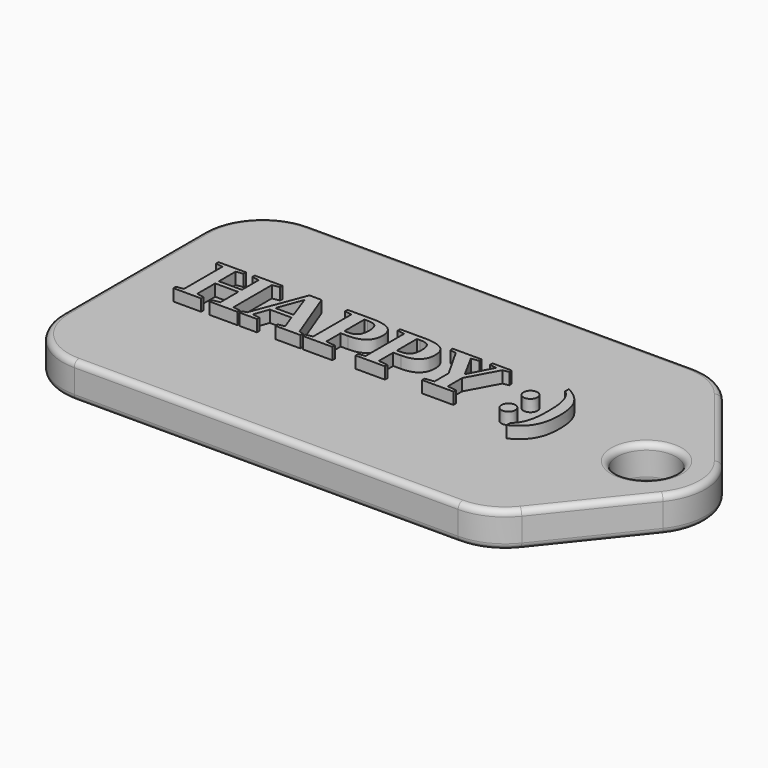
from build123d import *

# Parameters (mm, degrees)
F1_DEPTH     = 3
F2_R         = 5
F4_D         = 5
F5_R         = 5
F6_R         = 0.5
F7_TEXT_SIZE = 7.3078691558
F8_DEPTH     = 1


# Not quite as in the source:
# - Text() gives the source's letters only with a copy of the font that has no kerning and outlines rounded to 1/6400 em; it was checked with that copy


with BuildPart() as f1:
    # F0 (on Top) → F1 (new body)
    with BuildSketch(Plane.XY):
        Polygon((20, 12.5), (-20, 12.5), (-20, -12.5), (20, -12.5), (30, 0), align=None)
    extrude(amount=F1_DEPTH)

    # F2
    f2_edges = [f1.edges().sort_by_distance(p)[0] for p in [
        (30, 0, 1.5),
    ]]
    fillet(f2_edges, radius=F2_R)

    # F4 (through all)
    with Locations(Plane.XY.offset(3)):
        with Locations((23.5968757626, 0)):
            Hole(F4_D / 2)

    # F5
    f5_edges = [f1.edges().sort_by_distance(p)[0] for p in [
        (20, 12.5, 1.5),
        (-20, 12.5, 1.5),
        (-20, -12.5, 1.5),
        (20, -12.5, 1.5),
    ]]
    fillet(f5_edges, radius=F5_R)

    # F6
    f6_edges = [f1.edges().sort_by_distance(p)[0] for p in [
        (24.50122, -6.873475, 3),
        (19.762819, -12.006516, 3),
        (28.596876, 0, 3),
        (1.298438, -12.5, 3),
        (24.50122, 6.873475, 3),
        (-18.535534, -11.035534, 3),
        (19.762819, 12.006516, 3),
        (-20, 0, 3),
        (1.298438, 12.5, 3),
        (-18.535534, 11.035534, 3),
        (21.096876, 0, 3),
        (24.50122, -6.873475, 0),
        (19.762819, -12.006516, 0),
        (28.596876, 0, 0),
        (1.298438, -12.5, 0),
        (24.50122, 6.873475, 0),
        (-18.535534, -11.035534, 0),
        (19.762819, 12.006516, 0),
        (-20, 0, 0),
        (1.298438, 12.5, 0),
        (-18.535534, 11.035534, 0),
        (21.096876, 0, 0),
    ]]
    fillet(f6_edges, radius=F6_R)

    # F7 (on face) → F8 (join)
    with BuildSketch(Plane.XY.offset(3)):
        with Locations((-15.3254277539, -1.7268845113)):
            Text('HAPPY :)', F7_TEXT_SIZE, font='Tinos', font_style=FontStyle.BOLD, text_align=(TextAlign.LEFT, TextAlign.BOTTOM))
    extrude(amount=F8_DEPTH)


solid = f1.part
